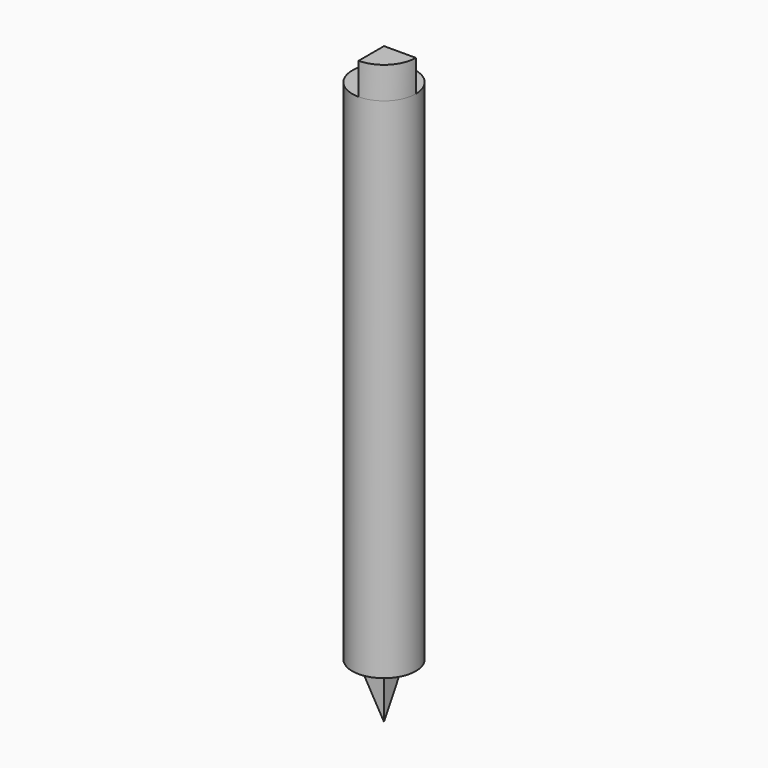
from build123d import *
from build123d import SkipClean  # not in build123d's __all__

# Parameters (mm, degrees)
F1_ANGLE = 90
F2_R     = 6.35
F3_DEPTH = 101.6
F5_DEPTH = 6.35


with BuildPart() as f1:
    # F0 (on Front) → F1 (revolve)
    with BuildSketch(Plane.XZ):
        Polygon((0, -10.9985226281), (0, 0), (-6.35, 0), align=None)
    revolve(axis=Axis((0, 0, -5.499261314), (0, 0, -1)), revolution_arc=F1_ANGLE)

    # F2 (on face) → F3 (join)
    with BuildSketch(Plane.XY):
        Circle(F2_R)
    extrude(amount=F3_DEPTH)

    # F4 (on face) → F5 (join)
    with BuildSketch(Plane.XY.offset(101.6)):
        with BuildLine():
            ThreePointArc((0, -6.35), (4.4901280605, -4.4901280605), (6.35, 0))
            Line((6.35, 0), (0, 0))
            Line((0, 0), (0, -6.35))
        make_face()
    with SkipClean():  # cleaning this boolean's faces spoils the solid; the shape is the same uncleaned
        extrude(amount=F5_DEPTH)


solid = f1.part
